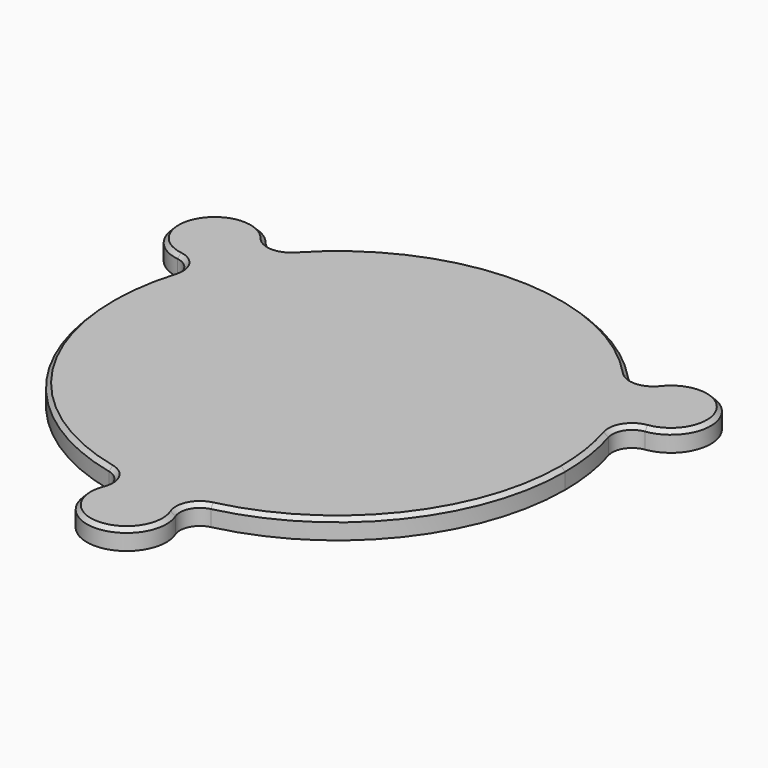
from build123d import *

# Parameters (mm, degrees)
F1_DEPTH = 5
F2_R     = 5
F3_SIZE  = 1


with BuildPart() as f1:
    # F0 (on Top) → F1 (new body)
    with BuildSketch(Plane.XY):
        with BuildLine():
            ThreePointArc((4.0489926269, -57.0063869992), (41.8181923846, -38.9533218826), (57.15, 0))
            ThreePointArc((57.15, 0), (55.6922778867, 12.8254701198), (51.3934756327, 24.996663025))
            ThreePointArc((51.3934756327, 24.996663025), (49.4933518263, 28.575), (47.3444830059, 32.0097239742))
            ThreePointArc((47.3444830059, 32.0097239742), (0, 57.15), (-47.3444830059, 32.0097239742))
            ThreePointArc((-47.3444830059, 32.0097239742), (-49.4933518263, 28.575), (-51.3934756327, 24.996663025))
            ThreePointArc((-51.3934756327, 24.996663025), (-49.4933518263, -28.575), (-4.0489926269, -57.0063869992))
            ThreePointArc((-4.0489926269, -57.0063869992), (0, -57.15), (4.0489926269, -57.0063869992))
        make_face()
        with BuildLine():
            ThreePointArc((47.3444830059, 32.0097239742), (49.4933518263, 28.575), (51.3934756327, 24.996663025))
            ThreePointArc((51.3934756327, 24.996663025), (65.9478344982, 38.075), (47.3444830059, 32.0097239742))
        make_face()
        with BuildLine():
            ThreePointArc((-51.3934756327, 24.996663025), (-49.4933518263, 28.575), (-47.3444830059, 32.0097239742))
            ThreePointArc((-47.3444830059, 32.0097239742), (-65.9478344982, 38.075), (-51.3934756327, 24.996663025))
        make_face()
        with BuildLine():
            ThreePointArc((-4.0489926269, -57.0063869992), (0, -76.15), (4.0489926269, -57.0063869992))
            ThreePointArc((4.0489926269, -57.0063869992), (0, -57.15), (-4.0489926269, -57.0063869992))
        make_face()
    extrude(amount=F1_DEPTH)

    # F2
    f2_edges = [f1.edges().sort_by_distance(p)[0] for p in [
        (51.393476, 24.996663, 2.5),
        (-4.048993, -57.006387, 2.5),
        (-47.344483, 32.009724, 2.5),
        (47.344483, 32.009724, 2.5),
        (-51.393476, 24.996663, 2.5),
        (4.048993, -57.006387, 2.5),
    ]]
    fillet(f2_edges, radius=F2_R)

    # F3
    f3_edges = [f1.edges().sort_by_distance(p)[0] for p in [
        (0, 57.15, 5),
        (45.702262, 37.347671, 5),
        (-45.702262, 37.347671, 5),
        (65.947834, 38.075, 5),
        (-65.947834, 38.075, 5),
        (55.195163, 20.905484, 5),
        (-55.195163, 20.905484, 5),
        (49.493352, -28.575, 5),
        (-49.493352, -28.575, 5),
        (9.492901, -58.253155, 5),
        (-9.492901, -58.253155, 5),
        (0, -76.15, 5),
    ]]
    chamfer(f3_edges, length=F3_SIZE)


solid = f1.part
